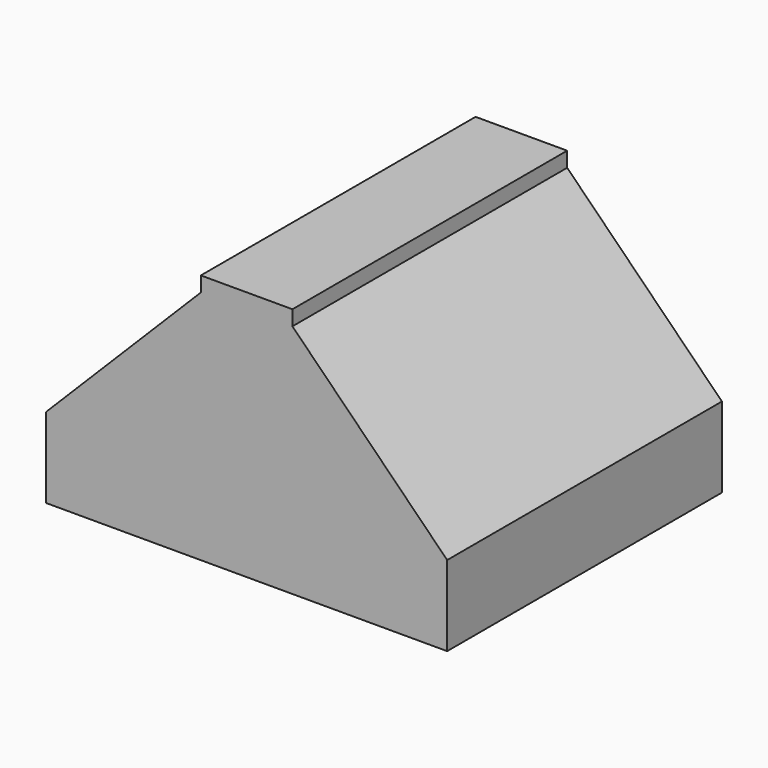
from build123d import *

# Parameters (mm, degrees)
F1_DEPTH = 66.5
F3_DEPTH = 2
F5_DEPTH = 2


with BuildPart() as f1:
    # F0 (on Front) → F1 (new body)
    with BuildSketch(Plane.XZ):
        Polygon((9.1355, 50), (0, 50), (-9.1355, 50), (-9.1355, 47), (-40, 16), (-40, 0), (0, 0), (40, 0), (40, 16), (9.1355, 47), align=None)
        Polygon((-6.7035206594, 44.8390617967), (0, 45.9953211248), (4.56775, 45.9953211248), (36.9867831469, 14.5120471716), (36.9867831469, 3.7666528951), (-36.0103435814, 3.7666528951), (-36.0103435814, 15.0574101135), align=None, mode=Mode.SUBTRACT)
    extrude(amount=F1_DEPTH)

    # F2 (on face) → F3 (join)
    with BuildSketch(Plane.XZ.offset(66.5)):
        Polygon((9.1355, 50), (-9.1355, 50), (-9.1355, 47), (-40, 16), (-40, 0), (40, 0), (40, 16), (9.1355, 47), align=None)
    extrude(amount=F3_DEPTH)

    # F4 (on face) → F5 (join)
    with BuildSketch(Plane(origin=(0, 0, 0), x_dir=(-1, 0, 0), z_dir=(0, 1, 0))):
        Polygon((9.1355, 50), (-9.1355, 50), (-9.1355, 47), (-40, 16), (-40, 0), (40, 0), (40, 16), (9.1355, 47), align=None)
    extrude(amount=-F5_DEPTH)


solid = f1.part
